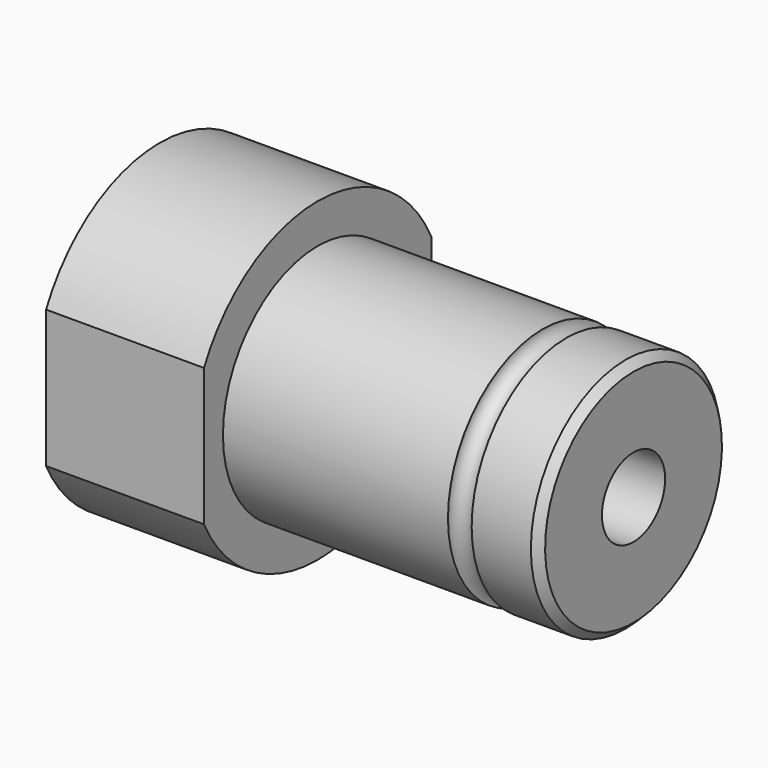
from build123d import *

# Parameters (mm, degrees)
F2_R     = 5
F3_DEPTH = 60.001
F4_SIZE  = 1
F5_R     = 1.5
F8_DEPTH = 20


with BuildPart() as f1:
    # F0 (on Front) → F1 (revolve)
    with BuildSketch(Plane.XZ):
        Polygon((0, 20), (0, 0), (60, 0), (60, 15), (20, 15), (20, 20), align=None)
    revolve(axis=Axis((31.1737104983, 0, 0), (-1, 0, 0)))

    # F2 (on face) → F3 (cut, through all)
    with BuildSketch(Plane.YZ.offset(60)):
        Circle(F2_R)
    extrude(amount=-F3_DEPTH, mode=Mode.SUBTRACT)

    # F4
    f4_edges = [f1.edges().sort_by_distance(p)[0] for p in [
        (60, 0, -15),
    ]]
    chamfer(f4_edges, length=F4_SIZE)

    # F5 (on Front) → F6 (revolve, cut)
    with BuildSketch(Plane.XZ):
        with Locations((50, 15)):
            Circle(F5_R)
    revolve(axis=Axis((31.1737104983, 0, 0), (-1, 0, 0)), mode=Mode.SUBTRACT)

    # F7 (on face) → F8 (cut, through all)
    with BuildSketch(Plane(origin=(0, 0, 0), x_dir=(0, -1, 0), z_dir=(-1, 0, 0))):
        with BuildLine():
            Line((18, 8.7177978871), (18, 42.813302379))
            Line((18, 42.813302379), (-18, 42.813302379))
            Line((-18, 42.813302379), (-18, 8.7177978871))
            ThreePointArc((-18, 8.7177978871), (0, 20), (18, 8.7177978871))
        make_face()
        with BuildLine():
            ThreePointArc((20, 0), (19.4935886896, 4.472135955), (18, 8.7177978871))
            Line((18, 8.7177978871), (18, -8.7177978871))
            ThreePointArc((18, -8.7177978871), (19.4935886896, -4.472135955), (20, 0))
        make_face()
        with BuildLine():
            Line((-18, -8.7177978871), (-18, 8.7177978871))
            ThreePointArc((-18, 8.7177978871), (-20, 0), (-18, -8.7177978871))
        make_face()
        with BuildLine():
            Line((18, -42.813302379), (18, -8.7177978871))
            ThreePointArc((18, -8.7177978871), (0, -20), (-18, -8.7177978871))
            Line((-18, -8.7177978871), (-18, -42.813302379))
            Line((-18, -42.813302379), (18, -42.813302379))
        make_face()
    extrude(amount=-F8_DEPTH, mode=Mode.SUBTRACT)


solid = f1.part
